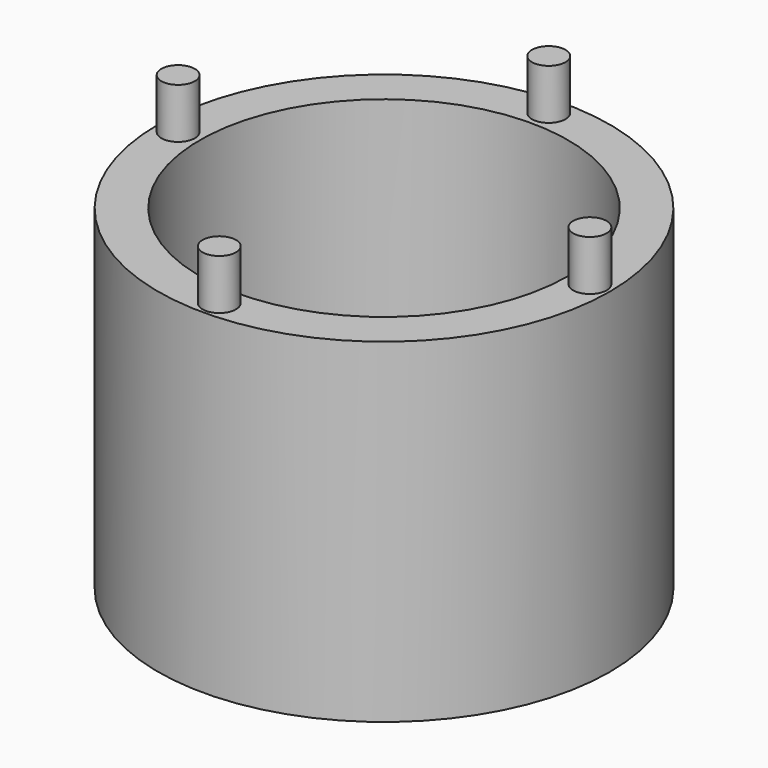
from build123d import *

# Parameters (mm, degrees)
F2_R     = 2.54
F3_DEPTH = 7.62
F4_D     = 5.08
F4_DEPTH = 34.291
F6_D     = 5.08
F6_DEPTH = 10.16
F6_TIP   = 1.5261859723
F8_DEPTH = 3.81


with BuildPart() as f1:
    # F0 (on Front) → F1 (revolve)
    with BuildSketch(Plane.XZ):
        Polygon((27.94, 20.2932615928), (27.94, 0), (34.29, 0), (34.29, 50.8), (27.94, 50.8), align=None)
    revolve(axis=Axis((0, 0, 10.1466307964), (0, 0, 1)))

    # F2 (on face) → F3 (join)
    with BuildSketch(Plane.XY.offset(50.8)):
        with Locations((0, 31.242)):
            Circle(F2_R)
        with Locations((31.242, 0)):
            Circle(F2_R)
        with Locations((0, -31.242)):
            Circle(F2_R)
        with Locations((-31.242, 0)):
            Circle(F2_R)
    extrude(amount=F3_DEPTH)

    # F4 (through all, one way)
    with BuildSketch(Plane.XZ):
        with Locations((0, 12.7)):
            Circle(F4_D / 2)
    extrude(amount=-F4_DEPTH, mode=Mode.SUBTRACT)

    # F6
    with Locations(Plane(origin=(0, 0, 0), x_dir=(1, 0, 0), z_dir=(0, 0, -1))):
        with Locations((0, 31.242), (31.242, 0), (0, -31.242), (-31.242, 0)):
            Hole(F6_D / 2, depth=F6_DEPTH)
            with Locations((0, 0, -(F6_DEPTH + F6_TIP / 2))):  # 118° drill point
                Cone(0, F6_D / 2, F6_TIP, mode=Mode.SUBTRACT)

    # F7 (on Top) → F8 (join)
    with BuildSketch(Plane.XY):
        with BuildLine():
            Line((0, 0), (-28.1686, 0))
            ThreePointArc((-28.1686, 0), (19.9182080765, -19.9182080765), (0, 28.1686))
            Line((0, 28.1686), (0, 0))
        make_face()
    extrude(amount=F8_DEPTH)


solid = f1.part
